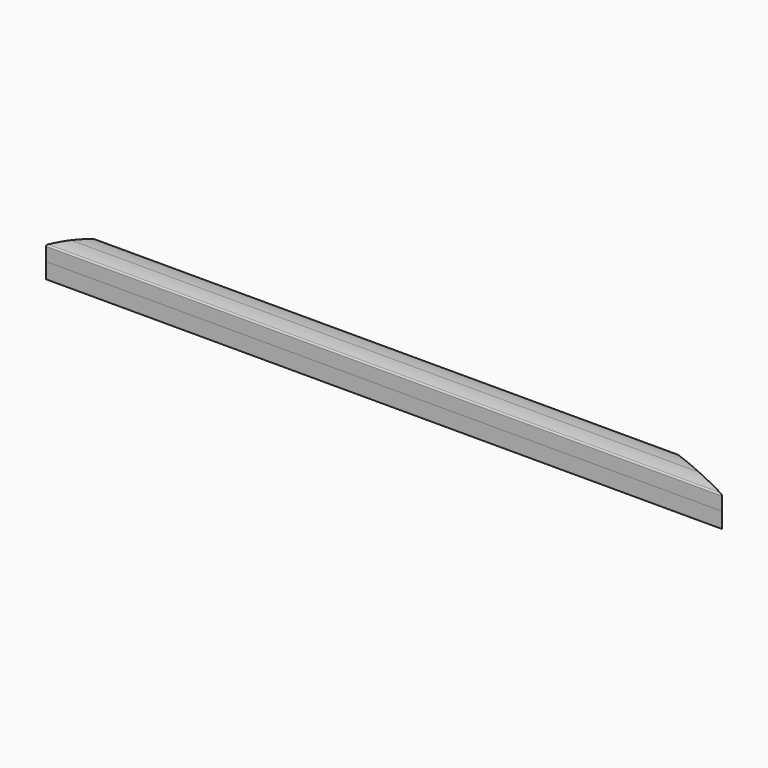
from build123d import *

# Parameters (mm, degrees)
F2_DEPTH      = 1000
F4_DEPTH      = 1000
F8_DEPTH      = 10.001
F8_DEPTH_BACK = 10.001


with BuildPart() as f2:
    # F1 (on Right) → F2 (new body)
    with BuildSketch(Plane.YZ):
        with BuildLine():
            Line((0, -9), (0, -10))
            Line((0, -10), (10, -10))
            Line((10, -10), (10, -0.2))
            Line((10, -0.2), (9, -0.2))
            ThreePointArc((9, -0.2), (8.5, -0.7), (9, -1.2))
            ThreePointArc((9, -1.2), (9.5, -1.7), (9, -2.2))
            Line((9, -2.2), (9, -9))
            Line((9, -9), (0, -9))
        make_face()
    extrude(amount=F2_DEPTH)

    # F5: F2 across plane


with BuildPart() as f4:
    # F3 (on Right) → F4 (new body)
    with BuildSketch(Plane.YZ):
        with BuildLine():
            Line((9, -0.2), (10, -0.2))
            Line((10, -0.2), (10, 8.1663783152))
            ThreePointArc((10, 8.1663783152), (9.7693092582, 8.8052548802), (9.1836734694, 9.1493656277))
            ThreePointArc((9.1836734694, 9.1493656277), (4.6114920912, 9.7868872364), (0, 10))
            Line((0, 10), (0, 9))
            ThreePointArc((0, 9), (4.5192622493, 8.7911494917), (9, 8.1663783152))
            Line((9, 8.1663783152), (9, 0.8))
            ThreePointArc((9, 0.8), (7.5, -0.7), (9, -2.2))
            ThreePointArc((9, -2.2), (9.5, -1.7), (9, -1.2))
            ThreePointArc((9, -1.2), (8.5, -0.7), (9, -0.2))
        make_face()
    extrude(amount=F4_DEPTH)

    # F6: F4 across plane


with BuildPart() as f2_1:
    add(f2.part)
    add(f2.part.mirror(Plane.XZ))


with BuildPart() as f4_1:
    add(f4.part)
    add(f4.part.mirror(Plane.XZ))


with BuildPart() as f8_tool:
    # F7 (on Top) → F8 (new body, two sides)
    with BuildSketch(Plane.XY) as f8_sk:
        Polygon((0, 10), (0, 0), (0, -10), (15.0710810021, 10), align=None)
        Polygon((379.4979817736, 10), (424, -10), (1016.9613361359, -10), (1016.9613361359, 10), (709.9114181152, 10), (424, 10), align=None)
    extrude(amount=F8_DEPTH)
    extrude(f8_sk.sketch, amount=-F8_DEPTH_BACK)


with BuildPart() as f2_2:
    add(f2_1.part)

    # F8: cut by f8_tool
    add(f8_tool.part, mode=Mode.SUBTRACT)


with BuildPart() as f4_2:
    add(f4_1.part)

    # F8: cut by f8_tool
    add(f8_tool.part, mode=Mode.SUBTRACT)


solid = Compound([f2_2.part, f4_2.part])
